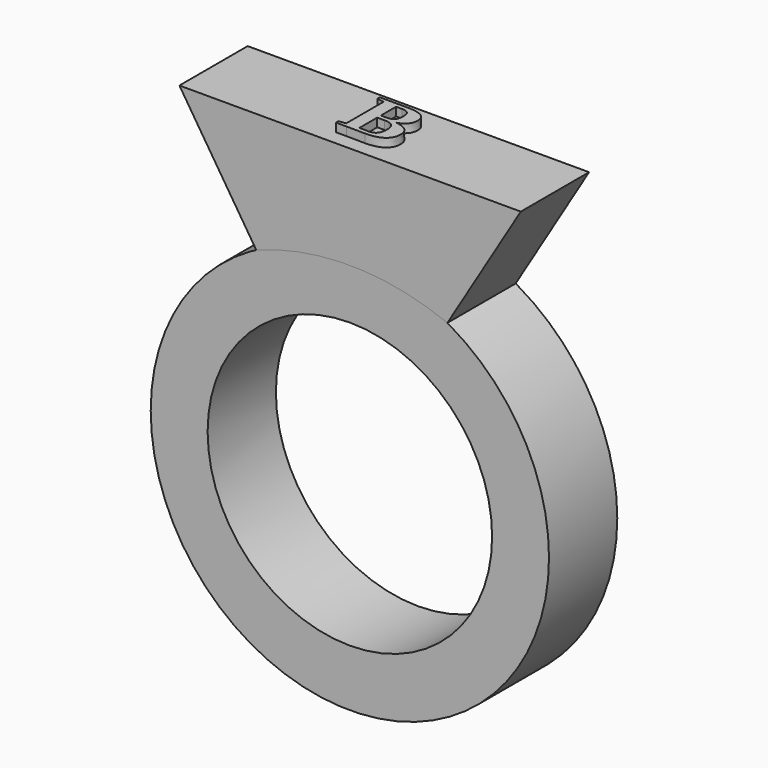
from build123d import *

# Parameters (mm, degrees)
F0_R         = 17.78
F0_R_2       = 12.7
F1_DEPTH     = 7.62
F3_DEPTH     = 7.62
F4_TEXT_SIZE = 7.4644691873
F5_DEPTH     = 0.762


# Not quite as in the source:
# - Text() gives the source's letters only with a copy of the font that has no kerning and outlines rounded to 1/6400 em; it was checked with that copy


with BuildPart() as f1:
    # F0 (on Front) → F1 (new body)
    with BuildSketch(Plane.XZ):
        Circle(F0_R)
        Circle(F0_R_2, mode=Mode.SUBTRACT)
    extrude(amount=F1_DEPTH)


with BuildPart() as f3:
    # F2 (on face) → F3 (new body)
    with BuildSketch(Plane(origin=(0, 0, 0), x_dir=(-1, 0, 0), z_dir=(0, 1, 0))):
        with BuildLine():
            Line((-15.260619137, 26.3805655804), (-8.706912157, 15.5021959958))
            ThreePointArc((-8.706912157, 15.5021959958), (-0.1896825481, 17.1957772458), (8.3628330405, 15.6904883142))
            Line((8.3628330405, 15.6904883142), (15.219380863, 26.3805655804))
            Line((15.219380863, 26.3805655804), (-15.260619137, 26.3805655804))
        make_face()
        with BuildLine():
            Line((-15.260619137, 26.3805655804), (-8.706912157, 15.5021959958))
            ThreePointArc((-8.706912157, 15.5021959958), (-0.1961150399, 17.7789183836), (8.3628330405, 15.6904883142))
            Line((8.3628330405, 15.6904883142), (15.219380863, 26.3805655804))
            Line((15.219380863, 26.3805655804), (-15.260619137, 26.3805655804))
        make_face()
    extrude(amount=-F3_DEPTH)

    # F4 (on face) → F5 (join)
    with BuildSketch(Plane.XY.offset(26.3805655804)):
        with Locations((-2.4080593139, -6.3170068897)):
            Text('B', F4_TEXT_SIZE, font='Tinos', font_style=FontStyle.BOLD, text_align=(TextAlign.LEFT, TextAlign.BOTTOM))
    extrude(amount=F5_DEPTH)


solid = Compound([f1.part, f3.part])
